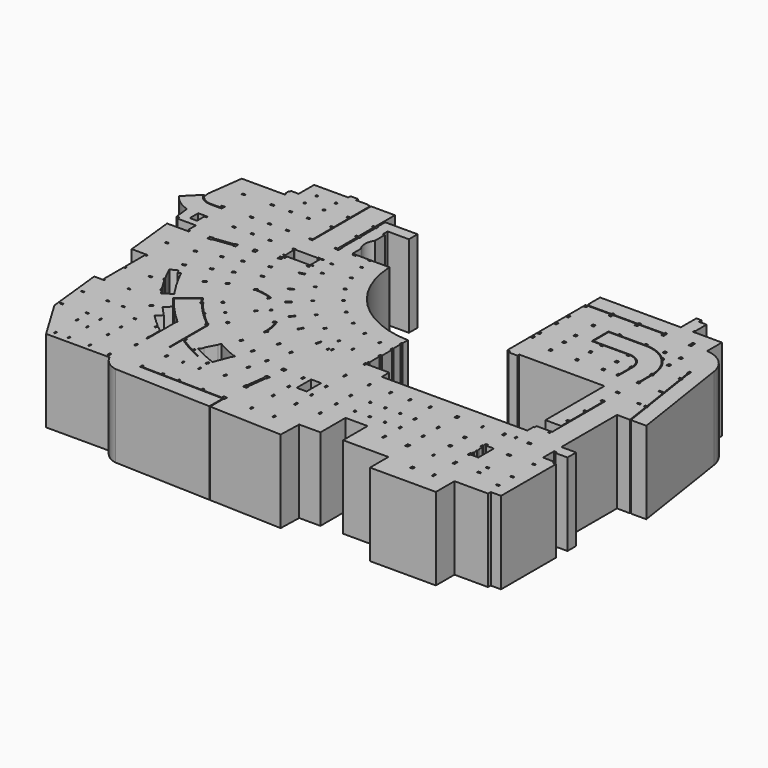
from build123d import *

# Parameters (mm, degrees)
F0_W     = 0.4
F0_H     = 0.8
F0_W_2   = 0.5
F0_H_2   = 0.9
F0_W_3   = 0.8
F0_H_3   = 0.4
F0_W_4   = 0.9
F0_H_4   = 0.5
F0_R     = 0.4
F0_H_5   = 1
F0_H_6   = 1.1
F0_W_5   = 2.99666
F0_H_7   = 5.520163
F0_R_2   = 0.35
F0_W_6   = 0.6
F0_H_8   = 0.6
F0_W_7   = 1.1
F0_H_9   = 0.800002
F0_W_8   = 0.799821
F0_W_9   = 1
F0_H_10  = 0.800178
F0_W_10  = 0.7
F0_H_11  = 0.7
F1_DEPTH = 25


# Not quite as in the source:
# - ends of sketch curves that miss each other by under 0.0002 mm in the source are joined


with BuildPart() as f1:
    # F0 (on Top) → F1 (new body)
    with BuildSketch(Plane.XY):
        with BuildLine():
            Line((-60.500308, -48.4425), (-41.219825, -48.4425))
            ThreePointArc((-41.219825, -48.4425), (-39.2824466185, -50.9328412394), (-36.4152879423, -52.2498967017))
            Line((-36.4152879423, -52.2498967017), (-7.058092, -53.288682))
            Line((-7.058092, -53.288682), (-7.058092, -48.1925))
            Line((-7.058092, -48.1925), (-32.583092, -47.6925))
            Line((-32.583092, -47.6925), (-32.583092, -46.7925))
            Line((-32.583092, -46.7925), (-32.083092, -46.7925))
            Line((-32.083092, -46.7925), (-32.083092, -47.442451))
            Line((-32.083092, -47.442451), (-26.308092, -47.556856))
            Line((-26.308092, -47.556856), (-26.308092, -46.91566))
            Line((-26.308092, -46.91566), (-25.808092, -46.91566))
            Line((-25.808092, -46.91566), (-25.808092, -47.566762))
            Line((-25.808092, -47.566762), (-21.258092, -47.656899))
            Line((-21.258092, -47.656899), (-21.258092, -47.014777))
            Line((-21.258092, -47.014777), (-20.758092, -47.014777))
            Line((-20.758092, -47.014777), (-20.758092, -47.666804))
            Line((-20.758092, -47.666804), (-13.958092, -47.801515))
            Line((-13.958092, -47.801515), (-13.958092, -47.158054))
            Line((-13.958092, -47.158054), (-13.458092, -47.158054))
            Line((-13.458092, -47.158054), (-13.458092, -47.811421))
            Line((-13.458092, -47.811421), (-7.608092, -47.927312))
            Line((-7.608092, -47.927312), (-7.602355, -47.1925))
            Line((-7.602355, -47.1925), (-6.558092, -47.1925))
            Line((-6.558092, -47.1925), (-6.558092, -48.1925))
            Line((-6.558092, -48.1925), (-6.808092, -48.1925))
            Line((-6.808092, -48.1925), (-6.808092, -53.297525))
            Line((-6.808092, -53.297525), (15.228774, -54.076935))
            Line((15.228774, -54.076935), (15.416908, -47.2925))
            Line((15.416908, -47.2925), (21.866908, -47.2925))
            Line((21.866908, -47.2925), (21.866908, -37.7675))
            Line((21.866908, -37.7675), (28.566908, -37.7675))
            Line((28.566908, -37.7675), (28.566908, -47.0925))
            Line((28.566908, -47.0925), (42.341908, -47.0925))
            Line((42.341908, -47.0925), (42.341908, -54.0825))
            Line((42.341908, -54.0825), (62.341908, -54.0825))
            Line((62.341908, -54.0825), (62.341908, -47.0175))
            Line((62.341908, -47.0175), (72.536908, -47.0175))
            Line((72.536908, -47.0175), (72.536908, -45.9975))
            Line((72.536908, -45.9975), (75.656908, -45.9975))
            Line((75.656908, -45.9975), (75.656908, -25.177417))
            Line((75.656908, -25.177417), (74.636908, -25.177417))
            Line((74.636908, -25.177417), (74.636908, -24.457417))
            Line((74.636908, -24.457417), (71.166908, -24.457417))
            Line((71.166908, -24.457417), (71.166908, -20.2425))
            Line((71.166908, -20.2425), (71.966908, -20.2425))
            Line((71.966908, -20.2425), (71.966908, -20.7925))
            Line((71.966908, -20.7925), (75.656908, -20.7925))
            Line((75.656908, -20.7925), (75.656908, -17.496517))
            Line((75.656908, -17.496517), (71.166908, -17.496517))
            Line((71.166908, -17.496517), (71.166908, 3.6075))
            Line((71.166908, 3.6075), (75.119187, 3.6075))
            Line((75.119187, 3.6075), (73.969052, 11.1075))
            Line((73.969052, 11.1075), (73.431908, 11.1075))
            Line((73.431908, 11.1075), (73.431908, 11.6075))
            Line((73.431908, 11.6075), (73.892376, 11.6075))
            Line((73.892376, 11.6075), (72.726906, 19.2075))
            Line((72.726906, 19.2075), (71.166908, 19.2075))
            Line((71.166908, 19.2075), (71.166908, 19.6075))
            Line((71.166908, 19.6075), (72.665566, 19.6075))
            Line((72.665566, 19.6075), (71.500043, 27.207842))
            Line((71.500043, 27.207842), (70.860716, 27.207842))
            Line((70.860716, 27.207842), (70.860716, 27.807842))
            Line((70.860716, 27.807842), (71.408032, 27.807842))
            Line((71.408032, 27.807842), (70.9672, 30.6825))
            Line((70.9672, 30.6825), (70.691908, 30.6825))
            Line((70.691908, 30.6825), (70.691908, 31.6825))
            Line((70.691908, 31.6825), (71.291908, 31.6825))
            Line((71.291908, 31.6825), (71.291908, 30.6825))
            Line((71.291908, 30.6825), (71.220122, 30.6825))
            Line((71.220122, 30.6825), (71.660955, 27.807842))
            Line((71.660955, 27.807842), (71.860716, 27.807842))
            Line((71.860716, 27.807842), (71.860716, 27.207842))
            Line((71.860716, 27.207842), (71.752966, 27.207842))
            Line((71.752966, 27.207842), (74.145299, 11.6075))
            Line((74.145299, 11.6075), (74.331908, 11.6075))
            Line((74.331908, 11.6075), (74.331908, 11.1075))
            Line((74.331908, 11.1075), (74.221975, 11.1075))
            Line((74.221975, 11.1075), (75.37211, 3.6075))
            Line((75.37211, 3.6075), (80.076468, 3.6075))
            Line((80.076468, 3.6075), (75.202936, 35.387673))
            ThreePointArc((75.202936, 35.387673), (72.5472354013, 40.3467347714), (67.3669079681, 42.5397344789))
            Line((67.3669079681, 42.5397344789), (67.366908, 48.1825))
            Line((67.366908, 48.1825), (67.350299, 48.1825))
            Line((67.350299, 48.1825), (58.591908, 48.1825))
            Line((58.591908, 48.1825), (58.591908, 48.6825))
            Line((58.591908, 48.6825), (58.791908, 48.6825))
            Line((58.791908, 48.6825), (58.791908, 53.0825))
            Line((58.791908, 53.0825), (56.491908, 53.0825))
            Line((56.491908, 53.0825), (56.491908, 54.0825))
            Line((56.491908, 54.0825), (54.89212, 54.0825))
            Line((54.89212, 54.0825), (54.891908, 48.1875))
            Line((54.891908, 48.1875), (30.391908, 48.1875))
            Line((30.391908, 48.1875), (30.391908, 43.7075))
            Line((30.391908, 43.7075), (30.841908, 43.7075))
            Line((30.841908, 43.7075), (30.841908, 43.2575))
            Line((30.841908, 43.2575), (37.741908, 43.2575))
            Line((37.741908, 43.2575), (37.741908, 43.7075))
            Line((37.741908, 43.7075), (38.441908, 43.7075))
            Line((38.441908, 43.7075), (38.441908, 43.2575))
            Line((38.441908, 43.2575), (45.741908, 43.2575))
            Line((45.741908, 43.2575), (45.741908, 43.7075))
            Line((45.741908, 43.7075), (46.441908, 43.7075))
            Line((46.441908, 43.7075), (46.441908, 43.2575))
            Line((46.441908, 43.2575), (53.741908, 43.2575))
            Line((53.741908, 43.2575), (53.741908, 43.7075))
            Line((53.741908, 43.7075), (54.441908, 43.7075))
            Line((54.441908, 43.7075), (54.441908, 43.0075))
            Line((54.441908, 43.0075), (30.091908, 43.005431))
            Line((30.091908, 43.005431), (30.091908, 13.3325))
            Line((30.091908, 13.3325), (30.941908, 13.3325))
            Line((30.941908, 13.3325), (30.941908, 12.6525))
            Line((30.941908, 12.6525), (33.716908, 12.6525))
            Line((33.716908, 12.6525), (33.716908, 13.3325))
            Line((33.716908, 13.3325), (59.586908, 13.322754))
            Line((59.586908, 13.322754), (59.586908, -9.084322))
            Line((59.586908, -9.084322), (64.366908, -9.084322))
            Line((64.366908, -9.084322), (64.366908, -6.2925))
            Line((64.366908, -6.2925), (63.616908, -6.2925))
            Line((63.616908, -6.2925), (63.616908, -5.6925))
            Line((63.616908, -5.6925), (64.366908, -5.6925))
            Line((64.366908, -5.6925), (64.366908, 0.1075))
            Line((64.366908, 0.1075), (63.616908, 0.1075))
            Line((63.616908, 0.1075), (63.616908, 0.7075))
            Line((63.616908, 0.7075), (64.366908, 0.7075))
            Line((64.366908, 0.7075), (64.366908, 6.8075))
            Line((64.366908, 6.8075), (63.616908, 6.8075))
            Line((63.616908, 6.8075), (63.616908, 7.4075))
            Line((63.616908, 7.4075), (64.616908, 7.407788))
            Line((64.616908, 7.407788), (64.616908, -12.7925))
            Line((64.616908, -12.7925), (59.866908, -12.7925))
            Line((59.866908, -12.7925), (59.866908, -13.6425))
            Line((59.866908, -13.6425), (59.586908, -13.6425))
            Line((59.586908, -13.6425), (59.586908, -15.9425))
            Line((59.586908, -15.9425), (15.416908, -15.9425))
            Line((15.416908, -15.9425), (15.416908, -13.142703))
            Line((15.416908, -13.142703), (8.456908, -13.142703))
            Line((8.456908, -13.142703), (8.456908, -13.7425))
            Line((8.456908, -13.7425), (7.956908, -13.7425))
            Line((7.956908, -13.7425), (7.956908, -12.8425))
            Line((7.956908, -12.8425), (8.196908, -12.8425))
            Line((8.196908, -12.8425), (8.196908, -11.9925))
            Line((8.196908, -11.9925), (8.476908, -11.9925))
            Line((8.476908, -11.9925), (8.476908, -8.2175))
            Line((8.476908, -8.2175), (8.096908, -8.2175))
            Line((8.096908, -8.2175), (8.096908, -7.3175))
            Line((8.096908, -7.3175), (8.646908, -7.315017))
            Line((8.646908, -7.315017), (8.646908, -3.6175))
            Line((8.646908, -3.6175), (8.196908, -3.6175))
            Line((8.196908, -3.6175), (8.196908, -2.8175))
            Line((8.196908, -2.8175), (8.476908, -2.8175))
            Line((8.476908, -2.8175), (8.476908, -0.1925))
            Line((8.476908, -0.1925), (8.196908, -0.1925))
            Line((8.196908, -0.1925), (8.196908, 0.6075))
            Line((8.196908, 0.6075), (8.476908, 0.6075))
            Line((8.476908, 0.6075), (8.476908, 2.600276))
            ThreePointArc((8.476908, 2.600276), (-9.9712627403, 10.438057178), (-18.2612355213, 28.6875000264))
            Line((-18.2612355213, 28.6875000264), (-18.303092, 28.6875))
            Line((-18.303092, 28.6875), (-18.303092, 29.0875))
            Line((-18.303092, 29.0875), (-29.513092, 29.1375))
            Line((-29.513092, 29.1375), (-29.513092, 32.239685))
            ThreePointArc((-29.513092, 32.239685), (-30.33307, 34.907532), (-29.5130925526, 37.5753793751))
            Line((-29.5130925526, 37.5753793751), (-29.513092, 41.3875))
            Line((-29.513092, 41.3875), (-30.133092, 41.3875))
            Line((-30.133092, 41.3875), (-30.133092, 43.2075))
            Line((-30.133092, 43.2075), (-23.682914, 43.2075))
            Line((-23.682914, 43.2075), (-23.682914, 46.5075))
            Line((-23.682914, 46.5075), (-33.513092, 46.5075))
            Line((-33.513092, 46.5075), (-33.513092, 43.5825))
            Line((-33.513092, 43.5825), (-33.233092, 43.5825))
            Line((-33.233092, 43.5825), (-33.233092, 42.7825))
            Line((-33.233092, 42.7825), (-33.383092, 42.7825))
            Line((-33.383092, 42.7825), (-33.383092, 37.2075))
            Line((-33.383092, 37.2075), (-33.233092, 37.2075))
            Line((-33.233092, 37.2075), (-33.233092, 36.4075))
            Line((-33.233092, 36.4075), (-33.383092, 36.4075))
            Line((-33.383092, 36.4075), (-33.383092, 29.9375))
            Line((-33.383092, 29.9375), (-33.233092, 29.9375))
            Line((-33.233092, 29.9375), (-33.233092, 28.2875))
            Line((-33.233092, 28.2875), (-33.633092, 28.2875))
            Line((-33.633092, 28.2875), (-33.633092, 28.4825))
            Line((-33.633092, 28.4825), (-34.583092, 28.4825))
            Line((-34.583092, 28.4825), (-34.583092, 28.9825))
            Line((-34.583092, 28.9825), (-33.933092, 28.9825))
            Line((-33.933092, 28.9825), (-33.933092, 36.4075))
            Line((-33.933092, 36.4075), (-34.583092, 36.4075))
            Line((-34.583092, 36.4075), (-34.583092, 36.9075))
            Line((-34.583092, 36.9075), (-33.983092, 36.9075))
            Line((-33.983092, 36.9075), (-33.983092, 42.7825))
            Line((-33.983092, 42.7825), (-34.583092, 42.7825))
            Line((-34.583092, 42.7825), (-34.583092, 43.28264))
            Line((-34.583092, 43.28264), (-33.982914, 43.282678))
            Line((-33.982914, 43.282678), (-33.983215, 50.7825))
            Line((-33.983215, 50.7825), (-41.233092, 50.7825))
            Line((-41.233092, 50.7825), (-41.233092, 28.647444))
            Line((-41.233092, 28.647444), (-41.233092, 28.4825))
            Line((-41.233092, 28.4825), (-42.333092, 28.4825))
            Line((-42.333092, 28.4825), (-42.333092, 28.9825))
            Line((-42.333092, 28.9825), (-41.483092, 28.9825))
            Line((-41.483092, 28.9825), (-41.483092, 36.4825))
            Line((-41.483092, 36.4825), (-42.333092, 36.4825))
            Line((-42.333092, 36.4825), (-42.333092, 36.9825))
            Line((-42.333092, 36.9825), (-41.483092, 36.9825))
            Line((-41.483092, 36.9825), (-41.483092, 42.7825))
            Line((-41.483092, 42.7825), (-42.333092, 42.7825))
            Line((-42.333092, 42.7825), (-42.333092, 43.2825))
            Line((-42.333092, 43.2825), (-41.483092, 43.2825))
            Line((-41.483092, 43.2825), (-41.483092, 50.7825))
            Line((-41.483092, 50.7825), (-42.333092, 50.7825))
            Line((-42.333092, 50.7825), (-42.333092, 51.0325))
            Line((-42.333092, 51.0325), (-46.033092, 51.0325))
            Line((-46.033092, 51.0325), (-46.033092, 51.811814))
            Line((-46.033092, 51.811814), (-48.311674, 51.811814))
            Line((-48.311674, 51.811814), (-48.311674, 50.9825))
            Line((-48.311674, 50.9825), (-58.658092, 50.9575))
            Line((-58.658092, 50.9575), (-58.658092, 45.1075))
            Line((-58.658092, 45.1075), (-60.983092, 45.1075))
            Line((-60.983092, 45.1075), (-60.983092, 44.6575))
            Line((-60.983092, 44.6575), (-61.283092, 44.6575))
            Line((-61.283092, 44.6575), (-61.283092, 43.4575))
            Line((-61.283092, 43.4575), (-60.983092, 43.4575))
            Line((-60.983092, 43.4575), (-60.983092, 42.7575))
            Line((-60.983092, 42.7575), (-74.065789, 42.7575))
            Line((-74.065789, 42.7575), (-75.49907, 31.910879))
            Line((-75.49907, 31.910879), (-75.294249, 30.037295))
            ThreePointArc((-75.294249, 30.037295), (-73.680373491, 28.6092623758), (-71.5907820068, 28.0824991741))
            Line((-71.5907820068, 28.0824991741), (-69.083092, 28.0825))
            Line((-69.083092, 28.0825), (-69.083092, 28.9825))
            Line((-69.083092, 28.9825), (-68.183092, 28.9825))
            Line((-68.183092, 28.9825), (-68.183092, 27.7825))
            Line((-68.183092, 27.7825), (-71.514599, 27.7825))
            ThreePointArc((-71.514599, 27.7825), (-73.9189967831, 28.3974531591), (-75.7056713657, 30.1199777782))
            Line((-75.7056713657, 30.1199777782), (-75.776699, 30.769697))
            Line((-75.776699, 30.769697), (-76.365067, 30.181151))
            Line((-76.365067, 30.181151), (-80.076467, 26.469751))
            ThreePointArc((-80.076467, 26.469751), (-77.6111300087, 24.002172522), (-74.4689289941, 22.4877740206))
            Line((-74.4689289941, 22.4877740206), (-73.973129, 17.9525))
            Line((-73.973129, 17.9525), (-73.174418, 17.9525))
            Line((-73.174418, 17.9525), (-73.174418, 17.2325))
            Line((-73.174418, 17.2325), (-67.558092, 17.2325))
            Line((-67.558092, 17.2325), (-67.558092, 14.2325))
            Line((-67.558092, 14.2325), (-66.908092, 14.2325))
            Line((-66.908092, 14.2325), (-66.908092, 13.7325))
            Line((-66.908092, 13.7325), (-73.508712, 13.733511))
            Line((-73.508712, 13.733511), (-71.883092, -1.172331))
            Line((-71.883092, -1.172331), (-71.893092, -1.7925))
            Line((-71.893092, -1.7925), (-66.908092, -1.7925))
            Line((-66.908092, -1.7925), (-66.908092, -2.2925))
            Line((-66.908092, -2.2925), (-67.458092, -2.2925))
            Line((-67.458092, -2.2925), (-67.458092, -9.8075))
            Line((-67.458092, -9.8075), (-66.908092, -9.8075))
            Line((-66.908092, -9.8075), (-66.908092, -10.3075))
            Line((-66.908092, -10.3075), (-67.458092, -10.3075))
            Line((-67.458092, -10.3075), (-67.458092, -17.9175))
            Line((-67.458092, -17.9175), (-66.908092, -17.9175))
            Line((-66.908092, -17.9175), (-66.908092, -18.3175))
            Line((-66.908092, -18.3175), (-70.008063, -18.3175))
            Line((-70.008063, -18.3175), (-68.098045, -35.789182))
            Line((-68.098045, -35.789182), (-60.500308, -48.4425))
        make_face()
        with Locations((-59.208092, -46.5175)):
            Rectangle(F0_W, F0_H, mode=Mode.SUBTRACT)
        with Locations((-55.108092, -46.5175)):
            Rectangle(F0_W, F0_H, mode=Mode.SUBTRACT)
        with Locations((-48.808092, -46.5175)):
            Rectangle(F0_W, F0_H, mode=Mode.SUBTRACT)
        with Locations((-42.233092, -47.2425)):
            Rectangle(F0_W_2, F0_H_2, mode=Mode.SUBTRACT)
        with Locations((-67.308092, -34.0175)):
            Rectangle(F0_W_3, F0_H_3, mode=Mode.SUBTRACT)
        with Locations((-55.108092, -39.5175)):
            Rectangle(F0_W, F0_H, mode=Mode.SUBTRACT)
        with Locations((-59.208092, -38.2175)):
            Rectangle(F0_W, F0_H, mode=Mode.SUBTRACT)
        with Locations((-59.608092, -34.0175)):
            Rectangle(F0_W_3, F0_H_3, mode=Mode.SUBTRACT)
        with Locations((-55.108092, -34.5175)):
            Rectangle(F0_W, F0_H, mode=Mode.SUBTRACT)
        with Locations((-48.808092, -39.5175)):
            Rectangle(F0_W, F0_H, mode=Mode.SUBTRACT)
        with Locations((-40.363092, -39.4675)):
            Rectangle(F0_W_2, F0_H_2, mode=Mode.SUBTRACT)
        with Locations((-48.808092, -34.5175)):
            Rectangle(F0_W, F0_H, mode=Mode.SUBTRACT)
        with Locations((-48.908092, -29.2175)):
            Rectangle(F0_W_3, F0_H_3, mode=Mode.SUBTRACT)
        with Locations((-31.108092, -39.4675)):
            Rectangle(F0_W_2, F0_H_2, mode=Mode.SUBTRACT)
        with Locations((-26.058092, -39.5175)):
            Rectangle(F0_W, F0_H, mode=Mode.SUBTRACT)
        with Locations((-21.008092, -39.5175)):
            Rectangle(F0_W, F0_H, mode=Mode.SUBTRACT)
        Polygon((-21.169261, -36.777247), (-21.635754, -36.597291), (-21.275843, -35.664304), (-20.809349, -35.84426), align=None, mode=Mode.SUBTRACT)
        with BuildLine():
            ThreePointArc((-20.6654099955, -35.0958009884), (-24.1828850835, -33.6141697841), (-27.6057386626, -31.9254023646))
            Line((-27.6057386626, -31.9254023646), (-27.371015, -31.483922))
            Line((-27.371015, -31.483922), (-27.238571, -31.554339))
            Line((-27.238571, -31.554339), (-27.194423, -31.577811))
            Line((-27.194423, -31.577811), (-26.724975, -30.694851))
            Line((-26.724975, -30.694851), (-26.901567, -30.600962))
            Line((-26.901567, -30.600962), (-25.19988, -27.400343))
            Line((-25.19988, -27.400343), (-25.310236, -27.34167))
            Line((-25.310236, -27.34167), (-24.840789, -26.458709))
            Line((-24.840789, -26.458709), (-24.399308, -26.693433))
            Line((-24.399308, -26.693433), (-24.457724, -26.803305))
            ThreePointArc((-24.457724, -26.803305), (-21.6876966437, -28.162915823), (-18.8462367659, -29.3661194013))
            Line((-18.8462367659, -29.3661194013), (-18.801451, -29.250023))
            Line((-18.801451, -29.250023), (-18.334958, -29.429979))
            Line((-18.334958, -29.429979), (-18.694869, -30.362965))
            Line((-18.694869, -30.362965), (-18.820116, -30.314649))
            Line((-18.820116, -30.314649), (-20.575393, -34.862569))
            Line((-20.575393, -34.862569), (-20.6654099955, -35.0958009884))
        make_face(mode=Mode.SUBTRACT)
        Polygon((-13.916253, -39.052429), (-14.400995, -38.929851), (-14.155838, -37.960367), (-13.671096, -38.082946), align=None, mode=Mode.SUBTRACT)
        Polygon((-6.169575, -40.474182), (-7.211093, -40.340991), (-7.084246, -39.34907), (-6.886025, -39.374418), (-6.140796, -33.546874), (-6.339017, -33.521526), (-6.21217, -32.529603), (-5.170651, -32.662793), (-5.297499, -33.654715), (-5.495867, -33.629339), (-6.240926, -39.456914), (-6.042727, -39.482259), align=None, mode=Mode.SUBTRACT)
        Polygon((-12.230798, -32.387227), (-12.71554, -32.264649), (-12.470384, -31.295169), (-11.985642, -31.417747), align=None, mode=Mode.SUBTRACT)
        Polygon((-5.641356, -28.065953), (-5.514509, -27.074031), (-5.018548, -27.137454), (-5.145395, -28.129377), align=None, mode=Mode.SUBTRACT)
        Polygon((-5.095781, -28.135721), (-4.968934, -27.143799), (-4.472991, -27.20722), (-4.599838, -28.199143), align=None, mode=Mode.SUBTRACT)
        with Locations((-67.308092, -26.0675)):
            Rectangle(F0_W_3, F0_H_3, mode=Mode.SUBTRACT)
        with Locations((-59.608092, -26.0675)):
            Rectangle(F0_W_3, F0_H_3, mode=Mode.SUBTRACT)
        with Locations((-54.958092, -26.0675)):
            Rectangle(F0_W_3, F0_H_3, mode=Mode.SUBTRACT)
        Polygon((-50.407666, -21.918406), (-50.618975, -21.465252), (-49.712667, -21.042634), (-49.501358, -21.495788), align=None, mode=Mode.SUBTRACT)
        with Locations((-59.608092, -18.1175)):
            Rectangle(F0_W_3, F0_H_3, mode=Mode.SUBTRACT)
        with Locations((-59.558092, -10.0575)):
            Rectangle(F0_W_4, F0_H_4, mode=Mode.SUBTRACT)
        with BuildLine():
            Line((-55.780314, -4.428994), (-54.981644, -4.056519))
            ThreePointArc((-54.981644, -4.056519), (-52.7891646239, -8.3201628324), (-50.2731386061, -12.4012457355))
            Line((-50.2731386061, -12.4012457355), (-49.57287, -13.422134))
            Line((-49.57287, -13.422134), (-52.162185, -15.254958))
            Line((-52.162185, -15.254958), (-52.865107, -14.231078))
            Line((-52.865107, -14.231078), (-52.972883, -14.070324))
            Line((-52.972883, -14.070324), (-53.206372, -14.224863))
            Line((-53.206372, -14.224863), (-53.647509, -13.557481))
            Line((-53.647509, -13.557481), (-53.4132088832, -13.4026096788))
            ThreePointArc((-53.4132088832, -13.4026096788), (-54.6659676321, -11.3987364029), (-55.8452486836, -9.3507603773))
            Line((-55.8452486836, -9.3507603773), (-56.09116, -9.484544))
            Line((-56.09116, -9.484544), (-56.47347, -8.781807))
            Line((-56.47347, -8.781807), (-56.227514, -8.648))
            ThreePointArc((-56.227514, -8.648), (-57.3228906469, -6.5108281364), (-58.3387659417, -4.3347419741))
            Line((-58.3387659417, -4.3347419741), (-56.270567, -3.351423))
            Line((-56.270567, -3.351423), (-55.780314, -4.428994))
        make_face(mode=Mode.SUBTRACT)
        Polygon((-57.487883, -0.745162), (-57.667839, -0.278669), (-56.734852, 0.081243), (-56.554897, -0.38525), align=None, mode=Mode.SUBTRACT)
        Polygon((-48.232262, -4.419644), (-48.466985, -3.978163), (-47.584025, -3.508716), (-47.349301, -3.950197), align=None, mode=Mode.SUBTRACT)
        Polygon((-43.375982, -1.837686), (-43.610699, -1.396202), (-42.727735, -0.92677), (-42.493018, -1.368254), align=None, mode=Mode.SUBTRACT)
        with BuildLine():
            Line((-40.213092, -35.4425), (-40.463092, -35.4425))
            Line((-40.463092, -35.4425), (-40.463092, -34.9175))
            Line((-40.463092, -34.9175), (-40.613092, -34.9175))
            Line((-40.613092, -34.9175), (-40.613092, -34.1175))
            Line((-40.613092, -34.1175), (-40.463092, -34.1175))
            Line((-40.463092, -34.1175), (-40.463092, -30.294089))
            Line((-40.463092, -30.294089), (-42.018985, -29.017353))
            Line((-42.018985, -29.017353), (-42.351459, -29.730345))
            Line((-42.351459, -29.730345), (-42.804612, -29.519035))
            Line((-42.804612, -29.519035), (-42.413727, -28.680778))
            ThreePointArc((-42.413727, -28.680778), (-44.3762006229, -26.9259036609), (-46.267212928, -25.0942489285))
            Line((-46.267212928, -25.0942489285), (-44.697613, -23.524649))
            Line((-44.697613, -23.524649), (-47.599817, -20.406109))
            Line((-47.599817, -20.406109), (-45.721493, -18.756258))
            ThreePointArc((-45.721493, -18.756258), (-47.1882101569, -17.0084933903), (-48.5900242638, -15.2082551978))
            Line((-48.5900242638, -15.2082551978), (-42.994458, -10.835328))
            ThreePointArc((-42.994458, -10.835328), (-42.3229150118, -11.7172914142), (-41.6338205102, -12.5856106032))
            ThreePointArc((-41.6338205102, -12.5856106032), (-41.2899844621, -12.73048424), (-41.2152664325, -13.0960371654))
            ThreePointArc((-41.2152664325, -13.0960371654), (-39.6365203712, -14.9158394193), (-37.9799756606, -16.6651196643))
            Line((-37.9799756606, -16.6651196643), (-37.737, -16.422144))
            Line((-37.737, -16.422144), (-37.312736, -16.846408))
            Line((-37.312736, -16.846408), (-37.555712, -17.089384))
            ThreePointArc((-37.555712, -17.089384), (-35.8064314193, -18.7459283712), (-33.9866289426, -20.3246749308))
            ThreePointArc((-33.9866289426, -20.3246749308), (-33.6210756112, -20.3993921577), (-33.4762022727, -20.7432289764))
            Line((-33.4762022727, -20.7432289764), (-33.258092, -20.919))
            Line((-33.258092, -20.919), (-33.258092, -29.411066))
            Line((-33.258092, -29.411066), (-32.538904, -29.880087))
            Line((-32.538904, -29.880087), (-32.921633, -30.466956))
            ThreePointArc((-32.921633, -30.466956), (-30.6873657923, -31.8545127154), (-28.3966103689, -33.1466826875))
            Line((-28.3966103689, -33.1466826875), (-28.068238, -32.529063))
            Line((-28.068238, -32.529063), (-27.626758, -32.763787))
            Line((-27.626758, -32.763787), (-27.955122, -33.381391))
            ThreePointArc((-27.955122, -33.381391), (-26.6074295798, -34.0703501601), (-25.2435059836, -34.7265909648))
            Line((-25.2435059836, -34.7265909648), (-25.370305, -34.998477))
            ThreePointArc((-25.370305, -34.998477), (-29.3929445563, -32.9438424909), (-33.2580923472, -30.6063685302))
            Line((-33.2580923472, -30.6063685302), (-33.258092, -35.4425))
            Line((-33.258092, -35.4425), (-33.508092, -35.4425))
            Line((-33.508092, -35.4425), (-33.508092, -21.038829))
            Line((-33.508092, -21.038829), (-33.580882, -20.980113))
            ThreePointArc((-33.580882, -20.980113), (-34.1283422784, -21.0180039329), (-34.1984198155, -20.4737271339))
            ThreePointArc((-34.1984198155, -20.4737271339), (-37.9491322926, -17.0585402926), (-41.3643192546, -13.3078282109))
            ThreePointArc((-41.3643192546, -13.3078282109), (-41.9085961946, -13.2377509591), (-41.8707036158, -12.6902904159))
            Line((-41.8707036158, -12.6902904159), (-43.041541, -11.189411))
            Line((-43.041541, -11.189411), (-48.242629, -15.254053))
            ThreePointArc((-48.242629, -15.254053), (-44.3141989442, -19.9507278746), (-39.9419218452, -24.2372778257))
            Line((-39.9419218452, -24.2372778257), (-40.209175, -24.534895))
            Line((-40.209175, -24.534895), (-40.213092, -35.4425))
        make_face(mode=Mode.SUBTRACT)
        Polygon((-22.728278, -22.48539), (-22.258846, -21.602426), (-21.817362, -21.837143), (-22.286794, -22.720107), align=None, mode=Mode.SUBTRACT)
        with Locations((-30.517702, -16.994638)):
            Circle(F0_R, mode=Mode.SUBTRACT)
        Polygon((-17.181849, -25.051584), (-16.821937, -24.118597), (-16.355444, -24.298553), (-16.715356, -25.23154), align=None, mode=Mode.SUBTRACT)
        Polygon((-11.367177, -26.932494), (-11.122021, -25.96301), (-10.637279, -26.085589), (-10.882436, -27.055072), align=None, mode=Mode.SUBTRACT)
        Polygon((-14.617479, -18.404055), (-14.257568, -17.471069), (-13.791075, -17.651025), (-14.150986, -18.584011), align=None, mode=Mode.SUBTRACT)
        Polygon((-9.135693, -20.147503), (-9.620434, -20.024924), (-9.375277, -19.055441), (-8.890536, -19.178019), align=None, mode=Mode.SUBTRACT)
        Polygon((-34.19794, -13.714359), (-34.622204, -13.290095), (-34.19794, -12.865831), (-33.773676, -13.290095), align=None, mode=Mode.SUBTRACT)
        with Locations((-37.88523, -9.62711)):
            Circle(F0_R, mode=Mode.SUBTRACT)
        with BuildLine():
            Line((-20.976393, -15.29162), (-20.739452, -14.888382))
            ThreePointArc((-20.739452, -14.888382), (-21.001284132, -12.4140755508), (-21.6575268171, -10.0140559337))
            Line((-21.6575268171, -10.0140559337), (-22.309812, -10.262443))
            Line((-22.309812, -10.262443), (-22.487746, -9.795175))
            Line((-22.487746, -9.795175), (-21.55321, -9.439307))
            ThreePointArc((-21.55321, -9.439307), (-20.8013420007, -11.8933117748), (-20.4568024587, -14.4366830245))
            Line((-20.4568024587, -14.4366830245), (-20.038784, -14.682888))
            Line((-20.038784, -14.682888), (-20.545304, -15.544922))
            Line((-20.545304, -15.544922), (-20.976393, -15.29162))
        make_face(mode=Mode.SUBTRACT)
        Polygon((-29.477266, -8.303831), (-28.840863, -7.667428), (-28.56097, -7.947349), (-29.194424, -8.586674), align=None, mode=Mode.SUBTRACT)
        with BuildLine():
            Line((-31.153035, -1.41922), (-30.904647, -0.766935))
            ThreePointArc((-30.904647, -0.766935), (-33.3046670889, -0.110692219), (-35.7789739905, 0.1511403845))
            Line((-35.7789739905, 0.1511403845), (-36.182211, -0.085801))
            Line((-36.182211, -0.085801), (-36.435514, 0.345288))
            Line((-36.435514, 0.345288), (-35.57348, 0.851808))
            Line((-35.57348, 0.851808), (-35.327275, 0.43379))
            ThreePointArc((-35.327275, 0.43379), (-32.7839037748, 0.0892499993), (-30.3298991007, -0.6626182532))
            Line((-30.3298991007, -0.6626182532), (-30.685767, -1.597154))
            Line((-30.685767, -1.597154), (-31.153035, -1.41922))
        make_face(mode=Mode.SUBTRACT)
        Polygon((-26.64881, -6.04106), (-26.931652, -5.758217), (-26.36596, -5.192525), (-26.083117, -5.475367), align=None, mode=Mode.SUBTRACT)
        Polygon((-20.9732, -5.7427), (-21.284529, -5.491554), (-20.78223, -4.868885), (-20.470901, -5.120031), align=None, mode=Mode.SUBTRACT)
        Polygon((-20.439507, -5.081114), (-20.750836, -4.829969), (-20.248537, -4.2073), (-19.937208, -4.458445), align=None, mode=Mode.SUBTRACT)
        Polygon((-15.642423, -9.264449), (-15.266866, -8.558083), (-14.913682, -8.745861), (-15.289239, -9.452228), align=None, mode=Mode.SUBTRACT)
        Polygon((-14.89021, -8.701713), (-15.243394, -8.513934), (-14.867836, -7.807566), (-14.514652, -7.995345), align=None, mode=Mode.SUBTRACT)
        Polygon((-7.641353, -12.4025), (-7.445228, -11.626916), (-7.057434, -11.724979), (-7.253559, -12.500562), align=None, mode=Mode.SUBTRACT)
        Polygon((-7.43297, -11.578442), (-7.236844, -10.802855), (-6.849051, -10.900918), (-7.045176, -11.676505), align=None, mode=Mode.SUBTRACT)
        Polygon((-3.639432, -13.199777), (-3.537954, -12.406239), (-3.141185, -12.456978), (-3.242663, -13.250516), align=None, mode=Mode.SUBTRACT)
        with Locations((-2.483092, -12.3925)):
            Rectangle(F0_W, F0_H, mode=Mode.SUBTRACT)
        Polygon((-4.019563, -8.351272), (-4.396944, -8.21867), (-4.131738, -7.463898), (-3.754357, -7.596499), align=None, mode=Mode.SUBTRACT)
        Polygon((-11.019306, -5.163089), (-10.623957, -4.467594), (-10.276213, -4.665266), (-10.671563, -5.360762), align=None, mode=Mode.SUBTRACT)
        Polygon((-16.684846, -1.233696), (-16.991839, -0.977269), (-16.475981, -0.365803), (-16.171997, -0.619716), align=None, mode=Mode.SUBTRACT)
        Polygon((-1.993938, -1.378371), (-1.728714, -0.6236), (-1.351335, -0.75621), (-1.61656, -1.510981), align=None, mode=Mode.SUBTRACT)
        with Locations((1.316908, -47.7425)):
            Rectangle(F0_W_2, F0_H_2, mode=Mode.SUBTRACT)
        with Locations((8.206908, -47.7425)):
            Rectangle(F0_W_2, F0_H_2, mode=Mode.SUBTRACT)
        with Locations((1.316908, -39.5175)):
            Rectangle(F0_W_2, F0_H_5, mode=Mode.SUBTRACT)
        with Locations((8.206908, -39.4675)):
            Rectangle(F0_W_2, F0_H_6, mode=Mode.SUBTRACT)
        with Locations((15.666908, -39.5675)):
            Rectangle(F0_W_2, F0_H_2, mode=Mode.SUBTRACT)
        with Locations((1.316908, -33.5425)):
            Rectangle(F0_W_2, F0_H_2, mode=Mode.SUBTRACT)
        with Locations((8.216908, -33.5425)):
            Rectangle(F0_W_2, F0_H_2, mode=Mode.SUBTRACT)
        with Locations((4.684928, -30.2038565)):
            Rectangle(F0_W_5, F0_H_7, mode=Mode.SUBTRACT)
        with Locations((1.216908, -28.0925)):
            Rectangle(F0_W_2, F0_H_2, mode=Mode.SUBTRACT)
        with Locations((8.216908, -28.0925)):
            Rectangle(F0_W_2, F0_H_2, mode=Mode.SUBTRACT)
        with Locations((15.666908, -33.5425)):
            Rectangle(F0_W_2, F0_H_2, mode=Mode.SUBTRACT)
        with Locations((15.666908, -28.0925)):
            Rectangle(F0_W_2, F0_H_2, mode=Mode.SUBTRACT)
        with Locations((35.091908, -39.5675)):
            Rectangle(F0_W_2, F0_H_6, mode=Mode.SUBTRACT)
        with Locations((21.462594, -33.693918)):
            Circle(F0_R_2, mode=Mode.SUBTRACT)
        with Locations((26.016908, -33.693918)):
            Rectangle(F0_W_6, F0_H_8, mode=Mode.SUBTRACT)
        with Locations((21.462594, -27.891082)):
            Circle(F0_R_2, mode=Mode.SUBTRACT)
        with Locations((26.016908, -27.891082)):
            Rectangle(F0_W_6, F0_H_8, mode=Mode.SUBTRACT)
        with Locations((30.571222, -33.693918)):
            Circle(F0_R_2, mode=Mode.SUBTRACT)
        with Locations((35.091908, -33.5425)):
            Rectangle(F0_W_2, F0_H_2, mode=Mode.SUBTRACT)
        with Locations((30.571222, -27.891082)):
            Circle(F0_R_2, mode=Mode.SUBTRACT)
        with Locations((35.091908, -27.8925)):
            Rectangle(F0_W_2, F0_H_2, mode=Mode.SUBTRACT)
        with Locations((50.241908, -47.7925)):
            Rectangle(F0_W_3, F0_H, mode=Mode.SUBTRACT)
        with Locations((56.591908, -47.6425)):
            Rectangle(F0_W_2, F0_H_6, mode=Mode.SUBTRACT)
        with Locations((71.616908, -42.1925)):
            Rectangle(F0_W_4, F0_H_4, mode=Mode.SUBTRACT)
        with Locations((42.241908, -39.6175)):
            Rectangle(F0_W_3, F0_H_5, mode=Mode.SUBTRACT)
        with Locations((50.091908, -39.7175)):
            Rectangle(F0_W, F0_H, mode=Mode.SUBTRACT)
        with Locations((56.541908, -39.5675)):
            Rectangle(F0_W_6, F0_H_6, mode=Mode.SUBTRACT)
        with Locations((42.091908, -33.5925)):
            Rectangle(F0_W_2, F0_H_5, mode=Mode.SUBTRACT)
        with Locations((42.091908, -27.9425)):
            Rectangle(F0_W_2, F0_H_5, mode=Mode.SUBTRACT)
        with Locations((50.191908, -33.4925)):
            Rectangle(F0_W_3, F0_H, mode=Mode.SUBTRACT)
        Polygon((56.241908, -28.4225), (56.241908, -27.4425), (56.841908, -27.4425), (56.841908, -28.0925), (59.166908, -28.0925), (59.166908, -33.9925), (56.841908, -33.9925), (56.841908, -34.3925), (56.241908, -34.3925), (56.241908, -33.2925), (56.591908, -33.2925), (56.591908, -32.6325), (56.741908, -32.6325), (56.741908, -31.7325), (56.591908, -31.7325), (56.591908, -31.3725), (56.741908, -31.3725), (56.741908, -30.4725), (56.591908, -30.4725), (56.591908, -29.2625), (55.991908, -29.2625), (55.991908, -28.4225), align=None, mode=Mode.SUBTRACT)
        with Locations((50.191908, -27.9425)):
            Rectangle(F0_W_3, F0_H, mode=Mode.SUBTRACT)
        with Locations((64.141908, -39.8425)):
            Rectangle(F0_W_4, F0_H_4, mode=Mode.SUBTRACT)
        with Locations((64.141908, -36.6925)):
            Rectangle(F0_W_4, F0_H_4, mode=Mode.SUBTRACT)
        with Locations((71.616908, -36.6925)):
            Rectangle(F0_W_4, F0_H_4, mode=Mode.SUBTRACT)
        with Locations((64.041908, -28.4425)):
            Rectangle(F0_W_7, F0_H_8, mode=Mode.SUBTRACT)
        with Locations((71.616908, -28.4925)):
            Rectangle(F0_W_4, F0_H_4, mode=Mode.SUBTRACT)
        with Locations((8.216908, -20.8925)):
            Rectangle(F0_W_2, F0_H_6, mode=Mode.SUBTRACT)
        with Locations((15.666908, -20.9925)):
            Rectangle(F0_W_2, F0_H_2, mode=Mode.SUBTRACT)
        with Locations((22.091908, -20.9925)):
            Rectangle(F0_W_2, F0_H_2, mode=Mode.SUBTRACT)
        with Locations((28.016908, -20.9925)):
            Rectangle(F0_W_2, F0_H_2, mode=Mode.SUBTRACT)
        with Locations((34.091908, -20.9425)):
            Rectangle(F0_W_2, F0_H_5, mode=Mode.SUBTRACT)
        with Locations((1.166908, -9.167501)):
            Rectangle(F0_W, F0_H_9, mode=Mode.SUBTRACT)
        Polygon((3.810122, -2.886268), (3.936537, -2.097521), (4.33169, -2.159619), (4.205081, -2.94957), align=None, mode=Mode.SUBTRACT)
        with Locations((42.241908, -20.9425)):
            Rectangle(F0_W_3, F0_H_5, mode=Mode.SUBTRACT)
        with Locations((50.091908, -21.0425)):
            Rectangle(F0_W, F0_H, mode=Mode.SUBTRACT)
        with Locations((56.541908, -20.8925)):
            Rectangle(F0_W_6, F0_H_6, mode=Mode.SUBTRACT)
        with Locations((59.716908, -20.427168)):
            Rectangle(F0_W, F0_H, mode=Mode.SUBTRACT)
        with Locations((64.041908, -20.7425)):
            Rectangle(F0_W_7, F0_H_8, mode=Mode.SUBTRACT)
        with Locations((64.216908, -13.2425)):
            Rectangle(F0_W_6, F0_H, mode=Mode.SUBTRACT)
        with Locations((-67.358092, 5.9575)):
            Rectangle(F0_W_4, F0_H_4, mode=Mode.SUBTRACT)
        Polygon((-51.073601, 1.72923), (-51.253557, 2.195723), (-50.320571, 2.555635), (-50.140615, 2.089141), align=None, mode=Mode.SUBTRACT)
        Polygon((-45.942176, 3.708743), (-46.122132, 4.175237), (-45.189145, 4.535148), (-45.00919, 4.068655), align=None, mode=Mode.SUBTRACT)
        Polygon((-59.820443, 6.489598), (-59.943022, 6.974339), (-58.973538, 7.219496), (-58.85096, 6.734755), align=None, mode=Mode.SUBTRACT)
        Polygon((-53.155241, 8.175053), (-53.277819, 8.659794), (-52.30834, 8.90495), (-52.185761, 8.420209), align=None, mode=Mode.SUBTRACT)
        Polygon((-47.823086, 9.523415), (-47.945664, 10.008156), (-46.976181, 10.253313), (-46.853602, 9.768572), align=None, mode=Mode.SUBTRACT)
        Polygon((-40.915517, 11.270158), (-41.038095, 11.7549), (-40.068612, 12.000057), (-39.946033, 11.515315), align=None, mode=Mode.SUBTRACT)
        Polygon((-71.033092, 19.2575), (-71.033092, 22.4575), (-68.183092, 22.4575), (-68.183092, 21.9575), (-68.833092, 21.9575), (-68.833092, 19.2575), align=None, mode=Mode.SUBTRACT)
        Polygon((-61.231615, 13.679546), (-61.365322, 14.720947), (-60.373405, 14.847794), (-60.347816, 14.649438), (-54.525397, 15.394011), (-54.550763, 15.592368), (-53.558841, 15.719215), (-53.425658, 14.677751), (-54.41758, 14.550904), (-54.442946, 14.749261), (-60.265046, 14.004729), (-60.239687, 13.806343), align=None, mode=Mode.SUBTRACT)
        Polygon((-48.956432, 15.249278), (-49.089615, 16.290742), (-48.097693, 16.417589), (-47.96451, 15.376125), align=None, mode=Mode.SUBTRACT)
        Polygon((-41.889101, 16.153051), (-41.952519, 16.648962), (-40.960611, 16.775831), (-40.897179, 16.279898), align=None, mode=Mode.SUBTRACT)
        with Locations((-59.983092, 22.2075)):
            Rectangle(F0_W_4, F0_H_4, mode=Mode.SUBTRACT)
        with Locations((-54.383092, 22.2075)):
            Rectangle(F0_W_4, F0_H_4, mode=Mode.SUBTRACT)
        with Locations((-48.983092, 22.2075)):
            Rectangle(F0_W_4, F0_H_4, mode=Mode.SUBTRACT)
        Polygon((-39.294648, 6.273113), (-39.474603, 6.739606), (-38.541617, 7.099518), (-38.361661, 6.633024), align=None, mode=Mode.SUBTRACT)
        Polygon((-26.382147, -0.393934), (-26.633293, -0.082605), (-26.010624, 0.419694), (-25.759479, 0.108364), align=None, mode=Mode.SUBTRACT)
        Polygon((-25.720562, 0.139758), (-25.971707, 0.451087), (-25.349038, 0.953387), (-25.097893, 0.642057), align=None, mode=Mode.SUBTRACT)
        Polygon((-29.448674, 5.623729), (-30.155043, 5.248171), (-30.342822, 5.601356), (-29.636453, 5.976913), align=None, mode=Mode.SUBTRACT)
        Polygon((-29.404526, 5.647202), (-29.592305, 6.000386), (-28.885937, 6.375943), (-28.698158, 6.022759), align=None, mode=Mode.SUBTRACT)
        Polygon((-21.867861, 3.898753), (-22.124288, 4.205747), (-21.510293, 4.718607), (-21.253866, 4.411613), align=None, mode=Mode.SUBTRACT)
        Polygon((-26.05368, 9.871288), (-26.251352, 10.219032), (-25.555857, 10.614381), (-25.358184, 10.266638), align=None, mode=Mode.SUBTRACT)
        Polygon((-12.069678, 4.292756), (-12.376665, 4.54919), (-11.863788, 5.163177), (-11.5568, 4.906743), align=None, mode=Mode.SUBTRACT)
        Polygon((-7.114658, 0.898054), (-7.461809, 1.096769), (-7.066432, 1.792276), (-6.719296, 1.593535), align=None, mode=Mode.SUBTRACT)
        Polygon((-16.55994, 8.85356), (-15.945953, 9.366415), (-15.689526, 9.059421), (-16.303513, 8.546567), align=None, mode=Mode.SUBTRACT)
        Polygon((-32.517506, 13.445368), (-33.293093, 13.249243), (-33.391155, 13.637036), (-32.615569, 13.833162), align=None, mode=Mode.SUBTRACT)
        Polygon((-32.469032, 13.457626), (-32.567094, 13.84542), (-31.791508, 14.041545), (-31.693445, 13.653752), align=None, mode=Mode.SUBTRACT)
        with BuildLine():
            Line((-42.183092, 21.9575), (-42.183092, 22.4575))
            Line((-42.183092, 22.4575), (-41.283092, 22.4575))
            Line((-41.283092, 22.4575), (-41.283092, 22.2075))
            Line((-41.283092, 22.2075), (-34.583092, 22.2075))
            Line((-34.583092, 22.2075), (-34.583092, 22.4575))
            Line((-34.583092, 22.4575), (-33.683092, 22.4575))
            Line((-33.683092, 22.4575), (-33.683092, 18.2075))
            Line((-33.683092, 18.2075), (-40.667784, 18.2075))
            Line((-40.667784, 18.2075), (-40.57516, 17.306946))
            Line((-40.57516, 17.306946), (-41.021836, 17.254694))
            Line((-41.021836, 17.254694), (-40.966944, 16.825446))
            Line((-40.966944, 16.825446), (-41.958867, 16.698604))
            Line((-41.958867, 16.698604), (-42.022284, 17.194515))
            Line((-42.022284, 17.194515), (-41.277114, 17.289808))
            Line((-41.277114, 17.289808), (-41.371307, 18.2075))
            Line((-41.371307, 18.2075), (-42.033092, 18.2075))
            Line((-42.033092, 18.2075), (-42.033092, 18.6075))
            Line((-42.033092, 18.6075), (-41.406688, 18.6075))
            ThreePointArc((-41.406688, 18.6075), (-41.5147896582, 20.2810263511), (-41.5573631308, 21.9574999992))
            Line((-41.5573631308, 21.9574999992), (-42.183092, 21.9575))
        make_face(mode=Mode.SUBTRACT)
        Polygon((-34.090369, 17.251161), (-34.143623, 17.647615), (-33.34757, 17.747251), (-33.296831, 17.352639), align=None, mode=Mode.SUBTRACT)
        with Locations((-33.233092, 18.4075)):
            Rectangle(F0_W_3, F0_H_3, mode=Mode.SUBTRACT)
        Polygon((-28.354487, 16.758857), (-29.10926, 16.493651), (-29.241861, 16.871033), (-28.487088, 17.136238), align=None, mode=Mode.SUBTRACT)
        Polygon((-22.26911, 18.897085), (-22.401711, 19.274466), (-21.646948, 19.539669), (-21.514347, 19.162287), align=None, mode=Mode.SUBTRACT)
        with Locations((-33.2331815, 22.2575)):
            Rectangle(F0_W_8, F0_H_3, mode=Mode.SUBTRACT)
        Polygon((-30.408092, 21.7075), (-30.408092, 22.107505), (-29.608095, 22.107505), (-29.599435, 22.109307), (-29.608095, 21.7075), align=None, mode=Mode.SUBTRACT)
        Polygon((-23.778186, 24.701429), (-23.841478, 25.09639), (-23.051557, 25.222976), (-22.988264, 24.828015), align=None, mode=Mode.SUBTRACT)
        Polygon((-19.750728, 13.454156), (-19.948401, 13.801899), (-19.252913, 14.197244), (-19.055241, 13.8495), align=None, mode=Mode.SUBTRACT)
        with Locations((-68.633092, 36.7325)):
            Rectangle(F0_W_4, F0_H_4, mode=Mode.SUBTRACT)
        with Locations((-59.883092, 28.7325)):
            Rectangle(F0_W_7, F0_H_4, mode=Mode.SUBTRACT)
        with Locations((-54.383092, 28.7325)):
            Rectangle(F0_W_4, F0_H_4, mode=Mode.SUBTRACT)
        with Locations((-48.983092, 28.7325)):
            Rectangle(F0_W_4, F0_H_4, mode=Mode.SUBTRACT)
        with Locations((-59.933092, 36.7325)):
            Rectangle(F0_W_9, F0_H_4, mode=Mode.SUBTRACT)
        with Locations((-54.433092, 36.7325)):
            Rectangle(F0_W_4, F0_H_4, mode=Mode.SUBTRACT)
        with Locations((-48.983092, 36.7325)):
            Rectangle(F0_W_4, F0_H_4, mode=Mode.SUBTRACT)
        with Locations((-54.58451, 42.353186)):
            Circle(F0_R_2, mode=Mode.SUBTRACT)
        with Locations((-54.58451, 46.9075)):
            Rectangle(F0_W_6, F0_H_8, mode=Mode.SUBTRACT)
        with Locations((-48.781674, 42.353186)):
            Circle(F0_R_2, mode=Mode.SUBTRACT)
        with Locations((-48.781674, 46.9075)):
            Rectangle(F0_W_6, F0_H_8, mode=Mode.SUBTRACT)
        with Locations((-28.658092, 28.8375)):
            Rectangle(F0_W_4, F0_H_4, mode=Mode.SUBTRACT)
        with Locations((-24.108092, 28.8875)):
            Rectangle(F0_W_3, F0_H_3, mode=Mode.SUBTRACT)
        with Locations((38.091908, 19.8075)):
            Rectangle(F0_W_3, F0_H, mode=Mode.SUBTRACT)
        with Locations((30.541908, 22.382678)):
            Rectangle(F0_W_3, F0_H, mode=Mode.SUBTRACT)
        with Locations((30.541908, 24.9325)):
            Rectangle(F0_W_3, F0_H, mode=Mode.SUBTRACT)
        with Locations((38.091908, 24.9325)):
            Rectangle(F0_W_3, F0_H, mode=Mode.SUBTRACT)
        with Locations((64.116908, 12.707678)):
            Rectangle(F0_W_9, F0_H_8, mode=Mode.SUBTRACT)
        with Locations((71.616908, 11.357159)):
            Rectangle(F0_W_4, F0_H_4, mode=Mode.SUBTRACT)
        with Locations((46.091908, 19.8075)):
            Rectangle(F0_W_3, F0_H, mode=Mode.SUBTRACT)
        with Locations((54.091908, 19.8075)):
            Rectangle(F0_W_3, F0_H, mode=Mode.SUBTRACT)
        with Locations((46.091908, 24.9325)):
            Rectangle(F0_W_3, F0_H, mode=Mode.SUBTRACT)
        with Locations((54.091908, 24.9325)):
            Rectangle(F0_W_3, F0_H, mode=Mode.SUBTRACT)
        with Locations((38.091908, 29.3075)):
            Rectangle(F0_W_3, F0_H, mode=Mode.SUBTRACT)
        with Locations((30.541908, 31.2825)):
            Rectangle(F0_W_3, F0_H, mode=Mode.SUBTRACT)
        with Locations((30.541908, 35.8575)):
            Rectangle(F0_W_3, F0_H, mode=Mode.SUBTRACT)
        with Locations((38.141908, 35.9575)):
            Rectangle(F0_W_3, F0_H, mode=Mode.SUBTRACT)
        with Locations((30.541908, 42.557589)):
            Rectangle(F0_W_3, F0_H_10, mode=Mode.SUBTRACT)
        with Locations((38.091908, 42.5575)):
            Rectangle(F0_W_3, F0_H, mode=Mode.SUBTRACT)
        with BuildLine():
            Line((42.828247, 29.4575), (42.828247, 35.8075))
            Line((42.828247, 35.8075), (45.691908, 35.8075))
            Line((45.691908, 35.8075), (45.691908, 36.3575))
            Line((45.691908, 36.3575), (46.491908, 36.3575))
            Line((46.491908, 36.3575), (46.491908, 35.8075))
            Line((46.491908, 35.8075), (53.691908, 35.8075))
            Line((53.691908, 35.8075), (53.691908, 36.3575))
            Line((53.691908, 36.3575), (54.491908, 36.3575))
            Line((54.491908, 36.3575), (54.491908, 35.800988))
            ThreePointArc((54.491908, 35.800988), (58.1148704221, 35.0402611589), (61.2680941562, 33.1007401768))
            Line((61.2680941562, 33.1007401768), (61.511548, 33.351813))
            Line((61.511548, 33.351813), (62.229464, 32.655683))
            Line((62.229464, 32.655683), (61.98601, 32.40461))
            ThreePointArc((61.98601, 32.40461), (64.0964809108, 29.1364374564), (64.9120168463, 25.3324999954))
            Line((64.9120168463, 25.3324999954), (65.166908, 25.3325))
            Line((65.166908, 25.3325), (65.166908, 24.5325))
            Line((65.166908, 24.5325), (64.916908, 24.5325))
            Line((64.916908, 24.5325), (64.916908, 20.2075))
            Line((64.916908, 20.2075), (65.166908, 20.2075))
            Line((65.166908, 20.2075), (65.166908, 19.4075))
            Line((65.166908, 19.4075), (64.366908, 19.4075))
            Line((64.366908, 19.4075), (64.366908, 20.2075))
            Line((64.366908, 20.2075), (64.666908, 20.2075))
            Line((64.666908, 20.2075), (64.666908, 24.5325))
            Line((64.666908, 24.5325), (64.366908, 24.5325))
            Line((64.366908, 24.5325), (64.366908, 25.3325))
            Line((64.366908, 25.3325), (64.661901, 25.3325))
            ThreePointArc((64.661901, 25.3325), (61.7429398974, 32.2976397449), (54.9162560061, 35.5271740807))
            Line((54.9162560061, 35.5271740807), (43.078247, 35.5575))
            Line((43.078247, 35.5575), (43.078247, 29.7075))
            Line((43.078247, 29.7075), (54.1169080003, 29.7075))
            ThreePointArc((54.1169080003, 29.7075), (54.1178605, 29.7075002561), (54.1188129997, 29.707499624))
            ThreePointArc((54.1188129997, 29.707499624), (57.3893160149, 28.3810902793), (58.8169080674, 25.1534700022))
            Line((58.8169080674, 25.1534700022), (58.816908, 19.4075))
            Line((58.816908, 19.4075), (58.216908, 19.4075))
            Line((58.216908, 19.4075), (58.216908, 20.4075))
            Line((58.216908, 20.4075), (58.566908, 20.4075))
            Line((58.566908, 20.4075), (58.566908, 24.332678))
            Line((58.566908, 24.332678), (58.216908, 24.332678))
            Line((58.216908, 24.332678), (58.216908, 25.332678))
            Line((58.216908, 25.332678), (58.555011, 25.332678))
            ThreePointArc((58.555011, 25.332678), (57.2811530749, 28.1364060558), (54.4919080241, 29.4416712847))
            Line((54.4919080241, 29.4416712847), (54.491908, 28.9075))
            Line((54.491908, 28.9075), (53.691908, 28.9075))
            Line((53.691908, 28.9075), (53.691908, 29.4575))
            Line((53.691908, 29.4575), (46.491908, 29.4575))
            Line((46.491908, 29.4575), (46.491908, 28.9075))
            Line((46.491908, 28.9075), (45.691908, 28.9075))
            Line((45.691908, 28.9075), (45.691908, 29.4575))
            Line((45.691908, 29.4575), (42.828247, 29.4575))
        make_face(mode=Mode.SUBTRACT)
        with Locations((59.991908, 35.7575)):
            Rectangle(F0_W_3, F0_H, mode=Mode.SUBTRACT)
        with Locations((64.816908, 31.2825)):
            Rectangle(F0_W_3, F0_H, mode=Mode.SUBTRACT)
        with Locations((64.816908, 35.8575)):
            Rectangle(F0_W_3, F0_H, mode=Mode.SUBTRACT)
        with Locations((46.091908, 42.5575)):
            Rectangle(F0_W_3, F0_H, mode=Mode.SUBTRACT)
        with Locations((54.091908, 42.5575)):
            Rectangle(F0_W_3, F0_H, mode=Mode.SUBTRACT)
        with Locations((62.491908, 42.5575)):
            Rectangle(F0_W_3, F0_H, mode=Mode.SUBTRACT)
        with Locations((62.441908, 43.3575)):
            Rectangle(F0_W_10, F0_H_11, mode=Mode.SUBTRACT)
    extrude(amount=F1_DEPTH)


solid = f1.part
